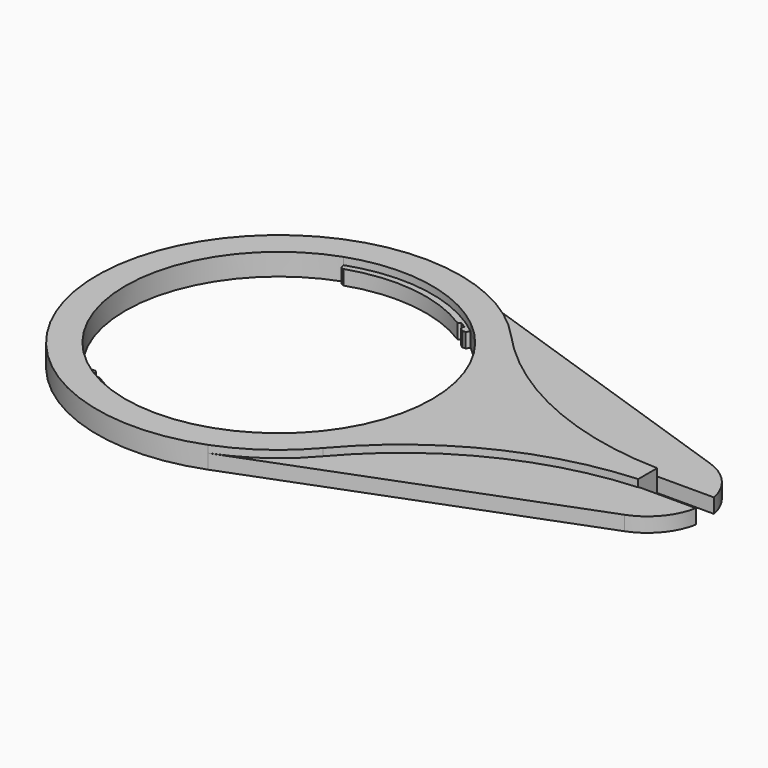
from build123d import *

# Parameters (mm, degrees)
F1_DEPTH    = 2
F3_DEPTH    = 1
F5_DEPTH    = 25
F6_T1_DEPTH = 3.532364341


# Not quite as in the source:
# - a fillet or chamfer that OpenCascade refuses, or shapes differently, is made with other operations: its cross-section is extruded or revolved along the edge and cut away or added


with BuildPart() as f1:
    # F0 (on Top) → F1 (new body)
    with BuildSketch(Plane.XY):
        with BuildLine():
            Line((56.2581913165, 7.0569766727), (11.7505642065, 22.2513897102))
            ThreePointArc((11.7505642065, 22.2513897102), (-21.3224604142, -1.8547742058), (12.5910944331, -24.7633510695))
            Line((12.5910944331, -24.7633510695), (56.5271609891, -7.9877403768))
            ThreePointArc((56.5271609891, -7.9877403768), (59.80596685, -5.6514457625), (61.5316564147, -2.0140241586))
            Line((61.5316564147, -2.0140241586), (53.6735452507, -2.0140241586))
            Line((53.6735452507, -2.0140241586), (53.6735452507, 1.1534155326))
            Line((53.6735452507, 1.1534155326), (61.4978499313, 1.1534155326))
            ThreePointArc((61.4978499313, 1.1534155326), (59.6568196422, 4.7964129612), (56.2581913165, 7.0569766727))
        make_face()
        with BuildLine():
            ThreePointArc((-9.6162715523, -17.7966343508), (-17.1193131366, 2.1791704159), (-3.3569313702, 18.4863852979))
            Line((-3.3569313702, 18.4863852979), (-3.0737131177, 17.6849569346))
            ThreePointArc((-3.0737131177, 17.6849569346), (7.1161082705, 18.5473361415), (16.4279902868, 14.3206339835))
            Line((16.4279902868, 14.3206339835), (16.9633620538, 14.9808438525))
            ThreePointArc((16.9633620538, 14.9808438525), (24.466403638, -4.9949609142), (10.7040218716, -21.3021757961))
            Line((10.7040218716, -21.3021757961), (10.4208036191, -20.5007474329))
            ThreePointArc((10.4208036191, -20.5007474329), (0.2309822309, -21.3631266398), (-9.0808997854, -17.1364244817))
            Line((-9.0808997854, -17.1364244817), (-9.6162715523, -17.7966343508))
        make_face(mode=Mode.SUBTRACT)
    extrude(amount=F1_DEPTH)

    # F2 (on face) → F3 (join)
    with BuildSketch(Plane.XY.offset(2)):
        with BuildLine():
            ThreePointArc((53.6735452507, 1.1654510324), (36.4234102314, 5.106684653), (22.0966452002, 15.4914949248))
            ThreePointArc((22.0966452002, 15.4914949248), (17.3479051946, 19.5208381125), (11.7505642065, 22.2513897102))
            ThreePointArc((11.7505642065, 22.2513897102), (-21.3224604142, -1.8547742058), (12.5910944331, -24.7633510695))
            ThreePointArc((12.5910944331, -24.7633510695), (18.1068462898, -21.8206319867), (22.7200407832, -17.6014435919))
            ThreePointArc((22.7200407832, -17.6014435919), (36.6180007946, -6.6981986771), (53.6735452507, -2.100107176))
            Line((53.6735452507, -2.100107176), (53.6735452507, -2.0140241586))
            Line((53.6735452507, -2.0140241586), (53.6735452507, 1.1534155326))
            Line((53.6735452507, 1.1534155326), (53.6735452507, 1.1654510324))
        make_face()
        with BuildLine():
            ThreePointArc((16.9633620538, 14.9808438525), (22.7211846654, 7.6694079147), (24.7735452507, -1.4078952491))
            ThreePointArc((24.7735452507, -1.4078952491), (20.9007484001, -13.591222859), (10.7040218716, -21.3021757961))
            ThreePointArc((10.7040218716, -21.3021757961), (0.0864795857, -22.2007536364), (-9.6162715523, -17.7966343508))
            ThreePointArc((-9.6162715523, -17.7966343508), (-17.1193131366, 2.1791704159), (-3.3569313702, 18.4863852979))
            ThreePointArc((-3.3569313702, 18.4863852979), (7.2606109157, 19.3849631382), (16.9633620538, 14.9808438525))
        make_face(mode=Mode.SUBTRACT)
    extrude(amount=F3_DEPTH)

    # F4 (on face) → F5 (cut)
    with BuildSketch(Plane(origin=(0, 0, 0), x_dir=(1, 0, 0), z_dir=(0, 0, -1))):
        Polygon((-8.5801632286, 17.98029692), (-8.4723387845, 17.2191802412), (-7.1583543904, 18.1015189737), (-7.951295166, 18.4884736217), align=None)
        Polygon((15.7582396641, -15.4063906521), (15.5428694561, -14.4470129162), (14.0254860744, -15.2497580275), (14.9163370952, -15.9154478461), align=None)
    extrude(amount=-F5_DEPTH, mode=Mode.SUBTRACT)

    # F6: chamfer of 0.3 on 4 edges, made by hand

    # F6_s2 → F6_t1 (cut)
    with BuildSketch(Plane.XY.offset(-0.7661821705)):
        with BuildLine():
            Line((-9.2684752215, -17.3677387978), (-8.8499270506, -17.3209446589))
            ThreePointArc((-8.8499270506, -17.3209446589), (-8.9624343354, -17.2317544465), (-9.0808997854, -17.1364244817))
            Line((-9.0808997854, -17.1364244817), (-9.2684752215, -17.3677387978))
        make_face()
        with BuildLine():
            Line((10.5200333329, -20.7815397421), (10.1413568327, -20.5972129374))
            ThreePointArc((10.1413568327, -20.5972129374), (10.2772447573, -20.5508744537), (10.4208036191, -20.5007474329))
            Line((10.4208036191, -20.5007474329), (10.5200333329, -20.7815397421))
        make_face()
        with BuildLine():
            Line((16.6155657229, 14.5519482995), (16.197017552, 14.5051541606))
            ThreePointArc((16.197017552, 14.5051541606), (16.3095248368, 14.4159639483), (16.4279902868, 14.3206339835))
            Line((16.4279902868, 14.3206339835), (16.6155657229, 14.5519482995))
        make_face()
        with BuildLine():
            Line((-2.7942663313, 17.7814224391), (-3.1729428315, 17.9657492438))
            Line((-3.1729428315, 17.9657492438), (-3.0737131177, 17.6849569346))
            ThreePointArc((-3.0737131177, 17.6849569346), (-2.9301542559, 17.7350839554), (-2.7942663313, 17.7814224391))
        make_face()
    extrude(amount=F6_T1_DEPTH, mode=Mode.SUBTRACT)


solid = f1.part
